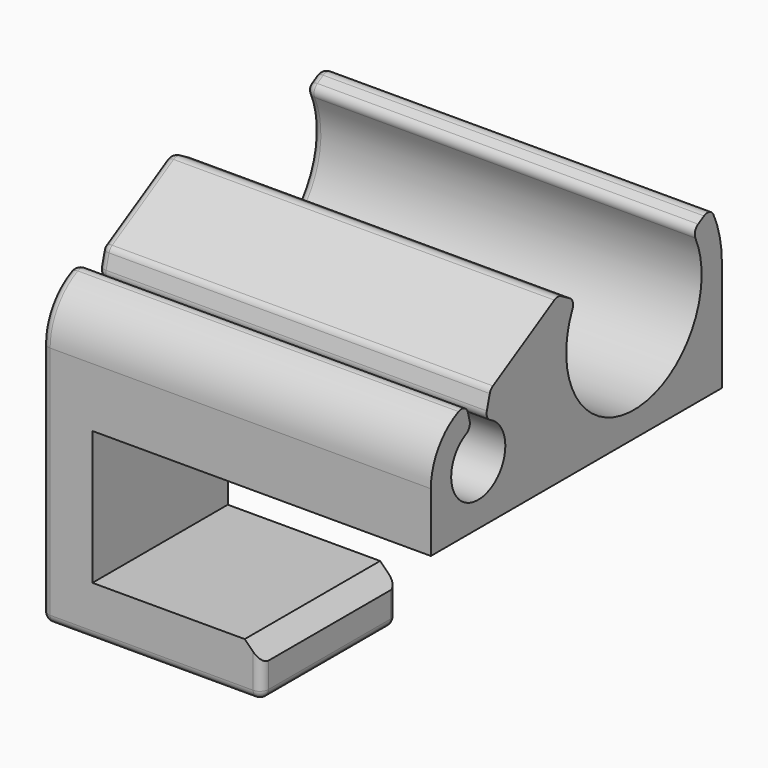
from build123d import *

# Parameters (mm, degrees)
F1_DEPTH    = 23
F3_DEPTH    = 10
F4_R        = 0.5
F5_T1_DEPTH = 14.1433659759


# Not quite as in the source:
# - a fillet or chamfer that OpenCascade refuses, or shapes differently, is made with other operations: its cross-section is extruded or revolved along the edge and cut away or added


with BuildPart() as f1:
    # F0 (on Right) → F1 (new body)
    with BuildSketch(Plane.YZ):
        with BuildLine():
            Line((-21.5, 0), (0, 0))
            Line((0, 0), (0, 6.5))
            ThreePointArc((0, 6.5), (-0.2214821291, 8.1823237932), (-0.8708348754, 9.75))
            Line((-0.8708348754, 9.75), (-2.1698729811, 9))
            ThreePointArc((-2.1698729811, 9), (-6.5, 1.5), (-10.8301270189, 9))
            Line((-10.8301270189, 9), (-12.1291651246, 9.75))
            Line((-12.1291651246, 9.75), (-17.0941333421, 6.880740392))
            Line((-17.0941333421, 6.880740392), (-17.4823619098, 5.4318516526))
            ThreePointArc((-17.4823619098, 5.4318516526), (-18, 1.5), (-18.5176380902, 5.4318516526))
            Line((-18.5176380902, 5.4318516526), (-18.9058666579, 6.880740392))
            ThreePointArc((-18.9058666579, 6.880740392), (-20.776736691, 5.6306650015), (-21.5, 3.5))
            Line((-21.5, 3.5), (-21.5, 0))
        make_face()
    extrude(amount=F1_DEPTH)

    # F2 (on face) → F3 (join)
    with BuildSketch(Plane.XZ.offset(21.5)):
        Polygon((3, 0), (0, 0), (0, -10.9), (13, -10.9), (13, -7.9), (3, -7.9), align=None)
    extrude(amount=-F3_DEPTH)

    # F4
    f4_edges = [f1.edges().sort_by_distance(p)[0] for p in [
        (0, -18, 1.5),
        (0, -17.288248, 6.156296),
        (0, -14.611649, 8.31537),
        (0, -11.479646, 9.375),
        (0, -6.5, 1.5),
        (0, -1.520354, 9.375),
        (0, 0, 3.25),
        (0, -5.75, 0),
        (0, -11.5, -5.45),
        (0, -16.5, -10.9),
        (0, -21.5, -3.7),
        (0, -18.711752, 6.156296),
        (6.5, -21.5, -10.9),
        (6.5, -11.5, -10.9),
        (13, -16.5, -10.9),
        (13, -11.5, -9.4),
        (13, -21.5, -9.4),
        (11.5, -17.482362, 5.431852),
        (11.5, -17.094133, 6.88074),
        (11.5, -18.517638, 5.431852),
        (11.5, -18.905867, 6.88074),
        (11.5, -12.129165, 9.75),
        (11.5, -10.830127, 9),
        (11.5, -2.169873, 9),
        (11.5, -0.870835, 9.75),
        (0, -20.776737, 5.630665),
        (0, -0.221482, 8.182324),
    ]]
    fillet(f4_edges, radius=F4_R)

    # F5: chamfer of 1 on 1 edges, made by hand

    # F5_s2 → F5_t1 (cut)
    with BuildSketch(Plane.XZ.offset(9.428317012)):
        Polygon((12, -7.9), (13, -8.9), (13, -7.9), align=None)
    extrude(amount=F5_T1_DEPTH, mode=Mode.SUBTRACT)


solid = f1.part
